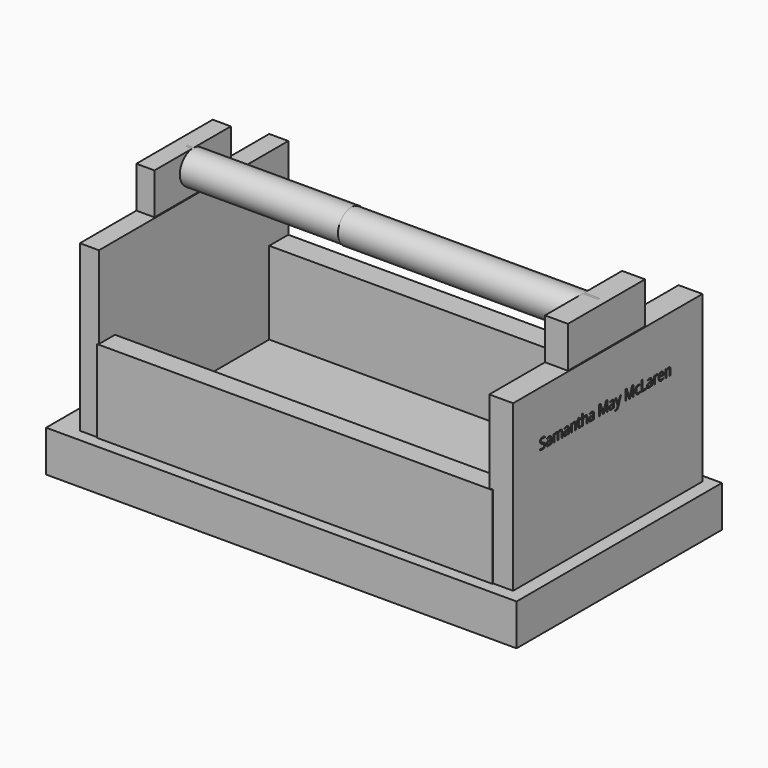
from build123d import *

# Parameters (mm, degrees)
F0_W          = 144.7520330548
F0_H          = 78.9823532104
F1_DEPTH      = 12.7
F2_W          = 121.5564757586
F2_H          = 6.4595229924
F2_H_2        = 7.3403622955
F3_DEPTH      = 25.4
F4_W          = 5.8722943068
F4_H          = 72.8164389729
F4_W_2        = 7.3403641582
F5_DEPTH      = 50.8
F6_W          = 5.5786818266
F6_H          = 29.3614678085
F6_W_2        = 7.046751678
F6_H_2        = 29.6550821513
F7_DEPTH      = 63.5
F8_R          = 5.08
F9_DEPTH      = 76.2
F10_R         = 5.08
F11_DEPTH     = 50.8
F12_TEXT_SIZE = 4.5228423571
F13_DEPTH     = 127


# Not quite as in the source:
# - Text() gives the source's letters only with a copy of the font that has no kerning and outlines rounded to 1/6400 em; it was checked with that copy


with BuildPart() as f1:
    # F0 (on Top) → F1 (new body)
    with BuildSketch(Plane.XY):
        with Locations((10.570127517, -3.6701858044)):
            Rectangle(F0_W, F0_H)
    extrude(amount=-F1_DEPTH)

    # F2 (on Top) → F3 (join)
    with BuildSketch(Plane.XY):
        with Locations((11.8913948536, -36.4082213491)):
            Rectangle(F2_W, F2_H)
        with Locations((11.8913948536, 29.8018911853)):
            Rectangle(F2_W, F2_H_2)
    extrude(amount=F3_DEPTH)

    # F4 (on Top) → F5 (join)
    with BuildSketch(Plane.XY):
        with Locations((-51.5293776989, -2.9361471534)):
            Rectangle(F4_W, F4_H)
        with Locations((75.1653574407, -2.9361471534)):
            Rectangle(F4_W_2, F4_H)
    extrude(amount=F5_DEPTH)

    # F6 (on Top) → F7 (join)
    with BuildSketch(Plane.XY):
        with Locations((-51.676183939, -2.9361471534)):
            Rectangle(F6_W, F6_H)
        with Locations((75.0185512006, -3.0829543248)):
            Rectangle(F6_W_2, F6_H_2)
    extrude(amount=F7_DEPTH)

    # F8 (on Right) → F9 (join)
    with BuildSketch(Plane.YZ):
        with Locations((-3.0829561874, 58.4293194115)):
            Circle(F8_R)
    extrude(amount=F9_DEPTH)

    # F10 (on Right) → F11 (join)
    with BuildSketch(Plane.YZ):
        with Locations((-2.7893420774, 58.4293194115)):
            Circle(F10_R)
    extrude(amount=-F11_DEPTH)

    # F12 (on Right) → F13 (cut)
    with BuildSketch(Plane.YZ):
        with Locations((-29.2675253566, 33.7613590614)):
            Text('Samantha May McLaren', F12_TEXT_SIZE, font='Open Sans', text_align=(TextAlign.LEFT, TextAlign.BOTTOM))
    extrude(amount=F13_DEPTH, mode=Mode.SUBTRACT)


solid = f1.part
